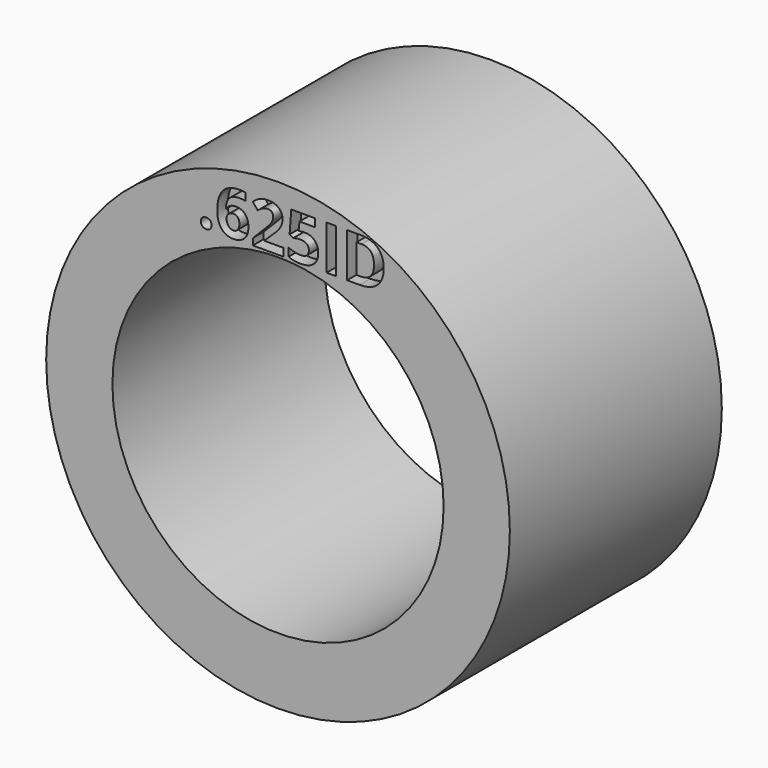
from build123d import *

# Parameters (mm, degrees)
F0_R         = 11.1125
F0_R_2       = 7.9375
F1_DEPTH     = 12.7
F2_TEXT_SIZE = 2.9660619071
F3_DEPTH     = 0.635


# Not quite as in the source:
# - Text() gives the source's letters only with a copy of the font that has no kerning and outlines rounded to 1/6400 em; it was checked with that copy


with BuildPart() as f1:
    # F0 (on Front) → F1 (new body)
    with BuildSketch(Plane.XZ):
        Circle(F0_R)
        Circle(F0_R_2, mode=Mode.SUBTRACT)
    extrude(amount=-F1_DEPTH)

    # F2 (on face) → F3 (cut)
    with BuildSketch(Plane.XZ):
        with Locations((-3.8632871583, 8.0355387181)):
            Text('.625ID', F2_TEXT_SIZE, font='Open Sans', font_style=FontStyle.BOLD, text_align=(TextAlign.LEFT, TextAlign.BOTTOM))
    extrude(amount=-F3_DEPTH, mode=Mode.SUBTRACT)


solid = f1.part
